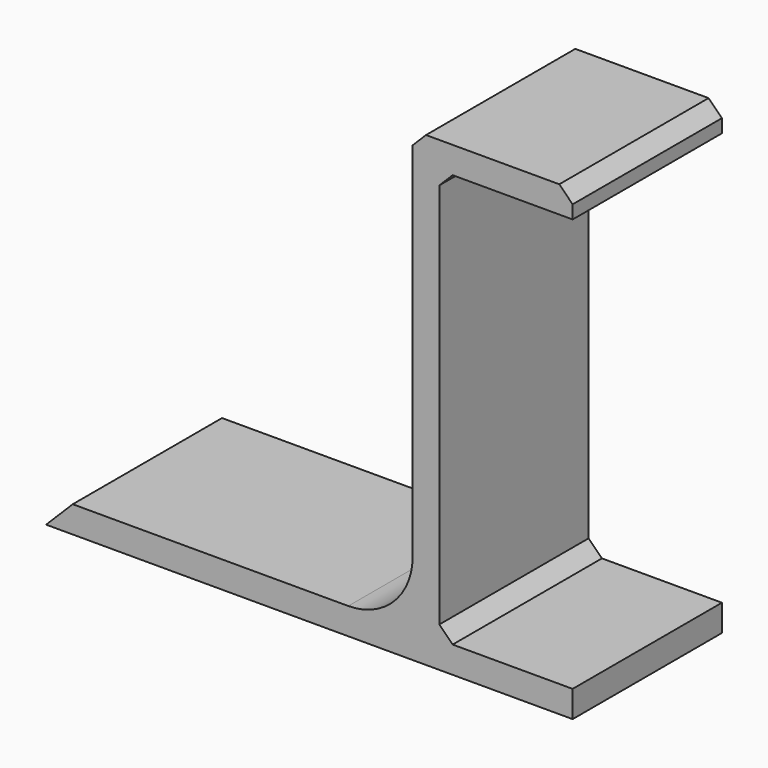
from build123d import *

# Parameters (mm, degrees)
F1_DEPTH    = 7
F2_R        = 2.4142135624
F3_SIZE     = 0.5
F4_T1_DEPTH = 13.4292074699


# Not quite as in the source:
# - a fillet or chamfer that OpenCascade refuses, or shapes differently, is made with other operations: its cross-section is extruded or revolved along the edge and cut away or added


with BuildPart() as f1:
    # F0 (on Front) → F1 (new body)
    with BuildSketch(Plane.XZ):
        Polygon((5, 0), (0, 0), (0, 15.5), (5, 15.5), (5, 16.5), (-1, 16.5), (-1, 1), (-1, 0), (-15, 0), (-15, -1), (5, -1), align=None)
    extrude(amount=F1_DEPTH)

    # F2
    f2_edges = [f1.edges().sort_by_distance(p)[0] for p in [
        (-1, -3.5, 0),
    ]]
    fillet(f2_edges, radius=F2_R)

    # F3
    f3_edges = [f1.edges().sort_by_distance(p)[0] for p in [
        (0, -3.5, 0),
        (0, -3.5, 15.5),
        (-1, -3.5, 16.5),
        (5, -3.5, 16.5),
    ]]
    chamfer(f3_edges, length=F3_SIZE)

    # F4: chamfer of 1.25 on 1 edges, made by hand

    # F4_s2 → F4_t1 (cut)
    with BuildSketch(Plane.XZ.offset(-3.214603735)):
        Polygon((-13.75, 0), (-15, -1.25), (-15, 0), align=None)
    extrude(amount=F4_T1_DEPTH, mode=Mode.SUBTRACT)


solid = f1.part
